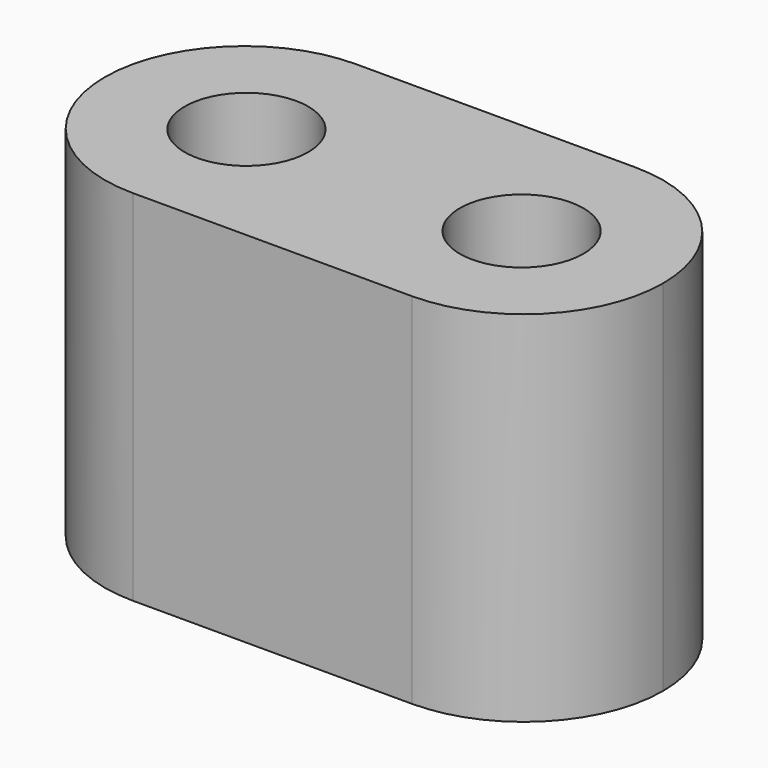
from build123d import *

# Parameters (mm, degrees)
F0_W     = 17.78
F0_H     = 8.89
F0_R     = 1.9685
F1_DEPTH = 11.43
F2_R     = 4.44499


# Not quite as in the source:
# - a fillet or chamfer is up to 0.001 mm smaller than in the source, because OpenCascade refuses the exact size


with BuildPart() as f1:
    # F0 (on Top) → F1 (new body)
    with BuildSketch(Plane.XY):
        with Locations((-118.9459740973, 32.9286159712)):
            Rectangle(F0_W, F0_H)
        with Locations((-123.3274740973, 32.9286159712)):
            Circle(F0_R, mode=Mode.SUBTRACT)
        with Locations((-114.5644740973, 32.9286159712)):
            Circle(F0_R, mode=Mode.SUBTRACT)
    extrude(amount=F1_DEPTH)

    # F2 (radius 4.445 in the source; OpenCascade refuses exactly that, so slightly less here)
    f2_edges = [f1.edges().sort_by_distance(p)[0] for p in [
        (-127.835974, 37.373616, 5.715),
        (-110.055974, 37.373616, 5.715),
        (-110.055974, 28.483616, 5.715),
        (-127.835974, 28.483616, 5.715),
    ]]
    fillet(f2_edges, radius=F2_R)


solid = f1.part
